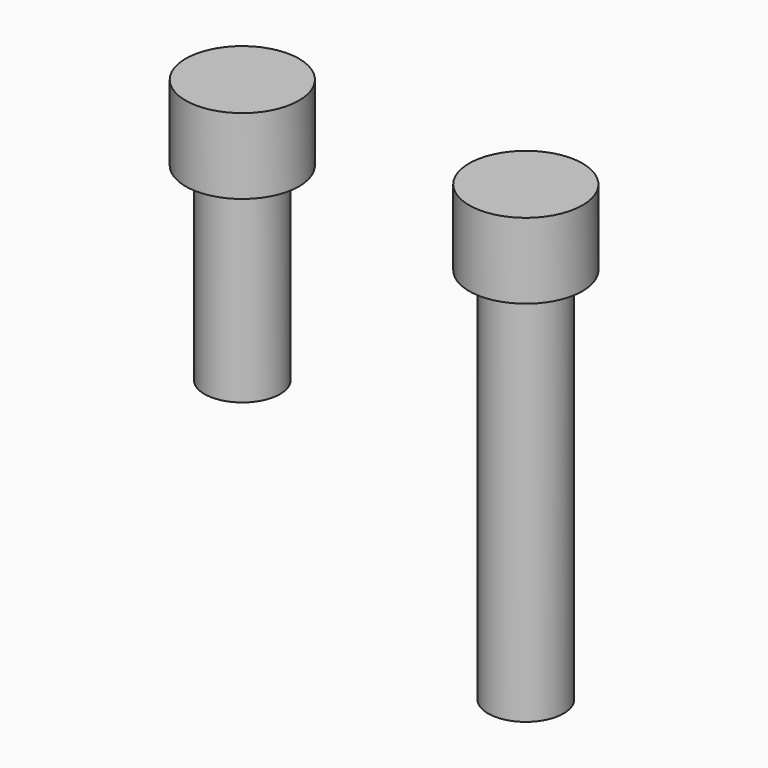
from build123d import *

# Parameters (mm, degrees)
F0_R     = 4
F1_DEPTH = 20
F2_R     = 6
F3_DEPTH = 8
F6_DEPTH = 20


# Not quite as in the source:
# - a feature of the source that left no trace in its solid (it failed there, or was rolled back) is left out


with BuildPart() as f1:
    # F0 (on Top) → F1 (new body)
    with BuildSketch(Plane.XY):
        Circle(F0_R)
    extrude(amount=F1_DEPTH)

    # F2 (on face) → F3 (join)
    with BuildSketch(Plane.XY.offset(20)):
        Circle(F2_R)
    extrude(amount=F3_DEPTH)


with BuildPart() as f5_1:
    # F5: copy of F1
    add(f1.part.moved(Location((30, 0, 0))))

    # F6 (add): a face of the model
    f6_faces = [f5_1.faces().sort_by_distance(p)[0] for p in [
        (30, 0, 0),
    ]]
    extrude(f6_faces, amount=F6_DEPTH)


solid = Compound([f1.part, f5_1.part])
